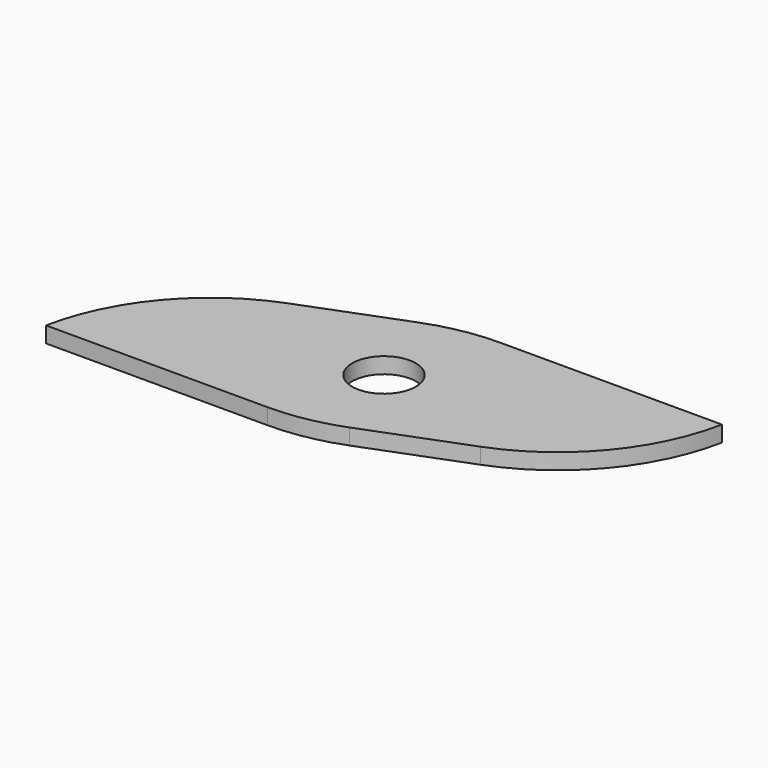
from build123d import *

# Parameters (mm, degrees)
F1_DEPTH    = 4
F2_R        = 8
F3_DEPTH    = 25
F4_T1_DEPTH = 50.4194138592
F4_T3_DEPTH = 170.6048746571


# Not quite as in the source:
# - a fillet or chamfer that OpenCascade refuses, or shapes differently, is made with other operations: its cross-section is extruded or revolved along the edge and cut away or added


with BuildPart() as f1:
    # F0 (on Top) → F1 (new body)
    with BuildSketch(Plane.XY):
        Polygon((65, 0), (65, 25), (0, 25), (-65, 0), (-65, -25), (0, -25), align=None)
    extrude(amount=F1_DEPTH)

    # F2 (on face) → F3 (cut)
    with BuildSketch(Plane.XY.offset(4)):
        Circle(F2_R)
    extrude(amount=-F3_DEPTH, mode=Mode.SUBTRACT)

    # F4: fillet of radius 50 on 4 edges, made by hand

    # F4_s2 → F4_t1 (cut)
    with BuildSketch(Plane.XY.offset(-23.2097069296)):
        with BuildLine():
            ThreePointArc((8.6650711936, -21.6672803102), (-0.1560137847, -24.1597600457), (-9.2838827718, -25))
            Line((-9.2838827718, -25), (0, -25))
            Line((0, -25), (8.6650711936, -21.6672803102))
        make_face()
        with BuildLine():
            ThreePointArc((9.2838827718, 25), (0.1560137847, 24.1597600457), (-8.6650711936, 21.6672803102))
            Line((-8.6650711936, 21.6672803102), (0, 25))
            Line((0, 25), (9.2838827718, 25))
        make_face()
    extrude(amount=F4_T1_DEPTH, mode=Mode.SUBTRACT)

    # F4_s4 → F4_t3 (cut)
    with BuildSketch(Plane.XY.offset(-83.3024373285)):
        with BuildLine():
            ThreePointArc((-33.9000144534, 11.9615329026), (-54.209630263, -2.5144156742), (-65, -25))
            Line((-65, -25), (-65, 0))
            Line((-65, 0), (-33.9000144534, 11.9615329026))
        make_face()
        with BuildLine():
            ThreePointArc((65, 25), (54.209630263, 2.5144156742), (33.9000144534, -11.9615329026))
            Line((33.9000144534, -11.9615329026), (65, 0))
            Line((65, 0), (65, 25))
        make_face()
    extrude(amount=F4_T3_DEPTH, mode=Mode.SUBTRACT)


solid = f1.part
